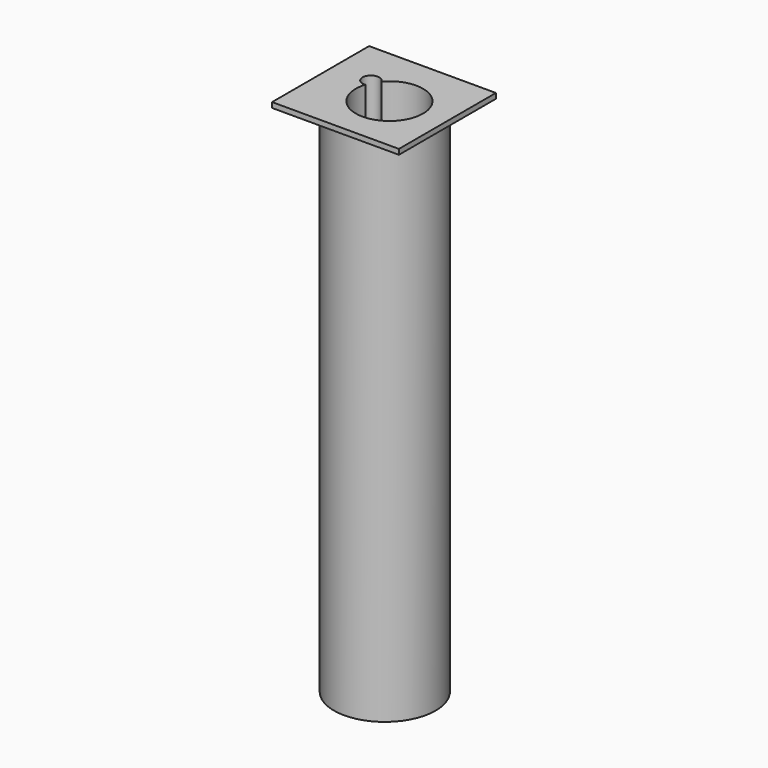
from build123d import *

# Parameters (mm, degrees)
F2_DEPTH  = 25.4
F3_R      = 248.0240216894
F4_DEPTH  = 2540
F5_W      = 119.7975315154
F5_H      = 181.1522692442
F5_W_2    = 320.4690925777
F5_H_2    = 205.2030339837
F5_W_3    = 6.3688382506
F5_W_4    = 172.1075996757
F6_DEPTH  = 25.4
F7_R      = 40.7896547179
F8_DEPTH  = 2565.401
F9_R      = 164.1580524022
F10_DEPTH = 2514.6


with BuildPart() as f2:
    # F1 (on face) → F2 (new body)
    with BuildSketch(Plane.XY):
        Polygon((-21.2495476007, -69.6708932519), (-21.2495476007, 53.5316392779), (0, 53.5316392779), (0, 76.628908515), (-80.3218334913, 76.628908515), (-80.3218334913, -69.6708932519), align=None)
        Polygon((0, 76.628908515), (0, 53.5316392779), (0, -69.6708932519), (74.5332688093, -69.6708932519), (74.5332688093, 76.628908515), align=None)
        Polygon((0, -69.6708932519), (-21.2495476007, -69.6708932519), (-80.3218334913, -69.6708932519), (-80.3218334913, -80.1510289311), (74.5332688093, -80.1510289311), (74.5332688093, -69.6708932519), align=None)
    extrude(amount=F2_DEPTH)

    # F3 (on Top) → F4 (join)
    with BuildSketch(Plane.XY):
        with Locations((-47.1228808165, 30.5453538895)):
            Circle(F3_R)
    extrude(amount=-F4_DEPTH)

    # F5 (on face) → F6 (join)
    with BuildSketch(Plane.XY):
        with Locations((36.0827576369, 215.6281396747)):
            Rectangle(F5_W, F5_H)
        with Locations((-184.0505544096, 215.6281396747)):
            Rectangle(F5_W_2, F5_H)
        with Locations((-184.0505544096, 22.4504880607)):
            Rectangle(F5_W_2, F5_H_2)
        with Locations((99.1659425199, 215.6281396747)):
            Rectangle(F5_W_3, F5_H)
        Polygon((95.9815233946, -80.1510289311), (-23.8160081208, -80.1510289311), (-23.8160081208, -285.3540629148), (102.3503616452, -285.3540629148), (102.3503616452, -80.1510289311), align=None)
        with Locations((-184.0505544096, -182.752545923)):
            Rectangle(F5_W_2, F5_H_2)
        with Locations((188.404161483, 215.6281396747)):
            Rectangle(F5_W_4, F5_H)
        with Locations((188.404161483, 22.4504880607)):
            Rectangle(F5_W_4, F5_H_2)
        with Locations((188.404161483, -182.752545923)):
            Rectangle(F5_W_4, F5_H_2)
    extrude(amount=F6_DEPTH)

    # F7 (on face) → F8 (cut, through all)
    with BuildSketch(Plane.XY.offset(25.4)):
        with Locations((-161.9917303324, 89.3510133028)):
            Circle(F7_R)
    extrude(amount=-F8_DEPTH, mode=Mode.SUBTRACT)

    # F9 (on face) → F10 (cut)
    with BuildSketch(Plane.XY.offset(25.4)):
        Circle(F9_R)
    extrude(amount=-F10_DEPTH, mode=Mode.SUBTRACT)


solid = f2.part
